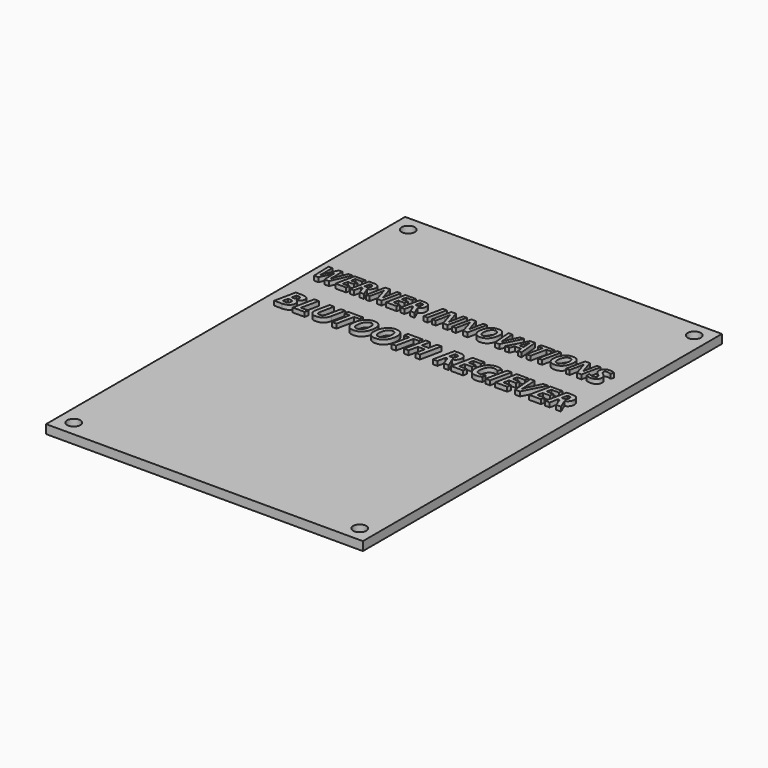
from build123d import *

# Parameters (mm, degrees)
F0_W         = 72
F0_H         = 102
F0_R         = 1.5
F1_DEPTH     = 2
F2_TEXT_SIZE = 6.0361828003
F4_DEPTH     = 1
F3_TEXT_SIZE = 6.7914335327
F5_DEPTH     = 1


# Not quite as in the source:
# - Text() gives the source's letters only with a copy of the font that has no kerning and outlines rounded to 1/6400 em; it was checked with that copy


with BuildPart() as f1:
    # F0 (on Top) → F1 (new body)
    with BuildSketch(Plane.XY):
        Rectangle(F0_W, F0_H)
        with Locations((-32.5, -47.5)):
            Circle(F0_R, mode=Mode.SUBTRACT)
        with Locations((32.5, -47.5)):
            Circle(F0_R, mode=Mode.SUBTRACT)
        with Locations((-32.5, 47.5)):
            Circle(F0_R, mode=Mode.SUBTRACT)
        with Locations((32.5, 47.5)):
            Circle(F0_R, mode=Mode.SUBTRACT)
    extrude(amount=F1_DEPTH)

    # F2 (on face) → F4 (join)
    with BuildSketch(Plane.XY.offset(2)):
        with Locations((-33.988004051, 21.7688333354)):
            Text('WERNER INNOVATIONS', F2_TEXT_SIZE, font='Open Sans', font_style=FontStyle.BOLDITALIC, text_align=(TextAlign.LEFT, TextAlign.BOTTOM))
    extrude(amount=F4_DEPTH)

    # F3 (on face) → F5 (join)
    with BuildSketch(Plane.XY.offset(2)):
        with Locations((-33, 9.834257315)):
            Text('BLUTOOTH RECIEVER', F3_TEXT_SIZE, font='Open Sans', font_style=FontStyle.BOLDITALIC, text_align=(TextAlign.LEFT, TextAlign.BOTTOM))
    extrude(amount=F5_DEPTH)


solid = f1.part
